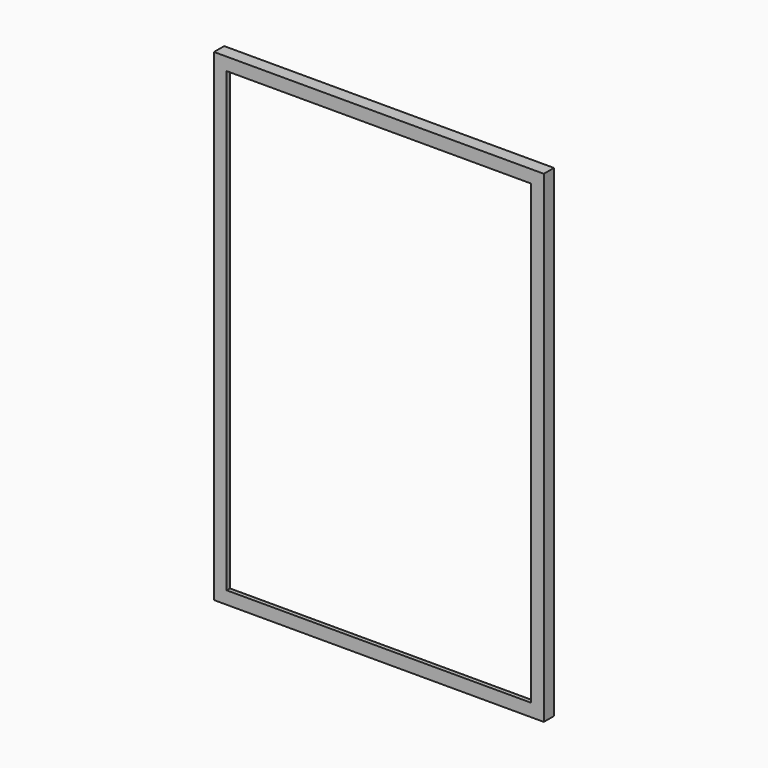
from build123d import *


with BuildPart() as f2:
    # F2: sweep along a path in F0
    with BuildLine(Plane.XZ) as f2_path:
        Line((263.9778585136, 299.2721299103), (263.9778585136, -615.1278700897))
        Line((263.9778585136, -615.1278700897), (-345.6221414864, -615.1278700897))
        Line((-345.6221414864, -615.1278700897), (-345.6221414864, 299.2721299103))
        Line((-345.6221414864, 299.2721299103), (263.9778585136, 299.2721299103))
    # F1 (on Top) → F2 (sweep)
    with BuildSketch(Plane.XY):
        with BuildLine():
            Line((288.2001969657, -12.7), (288.2001969657, 12.7))
            Line((288.2001969657, 12.7), (281.8501969657, 12.7))
            ThreePointArc((281.8501969657, 12.7), (277.3600689052, 10.8401280605), (275.5001969657, 6.35))
            ThreePointArc((275.5001969657, 6.35), (273.6403250262, 1.8598719395), (269.1501969657, 0))
            ThreePointArc((269.1501969657, 0), (264.6600689052, -1.8598719395), (262.8001969657, -6.35))
            Line((262.8001969657, -6.35), (262.8001969657, -12.7))
            Line((262.8001969657, -12.7), (288.2001969657, -12.7))
        make_face()
    sweep(path=f2_path.line, transition=Transition.RIGHT)


solid = f2.part
